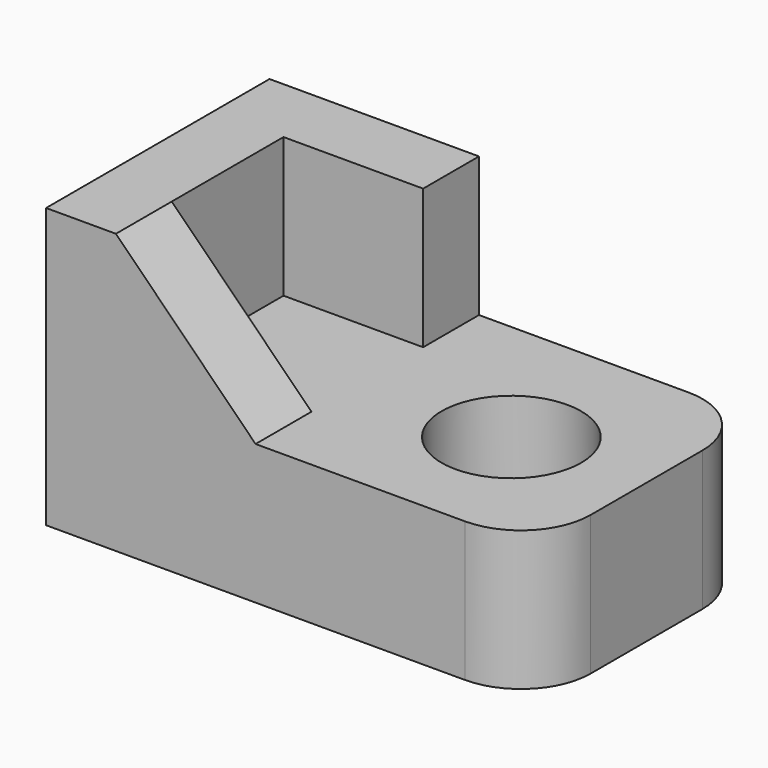
from build123d import *

# Parameters (mm, degrees)
F0_W     = 1778
F0_H     = 1016
F1_DEPTH = 1016
F3_DEPTH = 508
F6_DEPTH = 254
F4_W     = 508
F4_H     = 254
F7_DEPTH = 175.26
F8_R     = 254
F9_DEPTH = 508
F10_R    = 254
F11_R    = 254


with BuildPart() as f1:
    # F0 (on Top) → F1 (new body)
    with BuildSketch(Plane.XY):
        with Locations((889, 508)):
            Rectangle(F0_W, F0_H)
    extrude(amount=F1_DEPTH)

    # F2 (on face) → F3 (cut)
    with BuildSketch(Plane.XY.offset(1016)):
        Polygon((1778, 1016), (762, 1016), (762, 762), (254, 762), (254, 254), (762, 254), (762, 0), (1778, 0), align=None)
    extrude(amount=-F3_DEPTH, mode=Mode.SUBTRACT)

    # F5 (on face) → F6 (cut)
    with BuildSketch(Plane.XZ):
        Polygon((762, 1016), (253.9933919907, 1016), (762, 508), align=None)
    extrude(amount=-F6_DEPTH, mode=Mode.SUBTRACT)

    # F4 (on face) → F7 (cut)
    with BuildSketch(Plane.XY.offset(1016)):
        with Locations((508, 127)):
            Rectangle(F4_W, F4_H)
    extrude(amount=F7_DEPTH, mode=Mode.SUBTRACT)

    # F8 (on face) → F9 (cut)
    with BuildSketch(Plane.XY.offset(508)):
        with Locations((1302.4921417236, 487.4676764011)):
            Circle(F8_R)
    extrude(amount=-F9_DEPTH, mode=Mode.SUBTRACT)

    # F10
    f10_edges = [f1.edges().sort_by_distance(p)[0] for p in [
        (1778, 0, 254),
    ]]
    fillet(f10_edges, radius=F10_R)

    # F11
    f11_edges = [f1.edges().sort_by_distance(p)[0] for p in [
        (1778, 1016, 254),
    ]]
    fillet(f11_edges, radius=F11_R)


solid = f1.part
